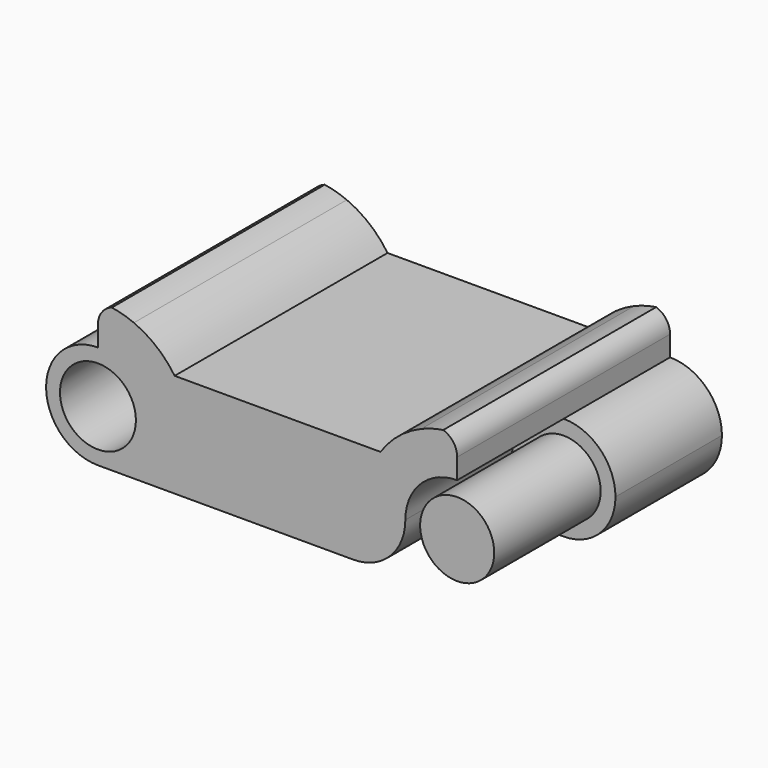
from build123d import *

# Parameters (mm, degrees)
F1_DEPTH = 14.37
F0_R     = 2
F2_DEPTH = 7.185
F3_R     = 2.05
F4_DEPTH = 7.185


with BuildPart() as f1:
    # F0 (on Front) → F1 (new body)
    with BuildSketch(Plane.XZ):
        with BuildLine():
            ThreePointArc((7.1321428571, 0.3034947896), (7.7481620558, 0.0769305381), (8.4, 0))
            Line((8.4, 0), (16.6, 0))
            ThreePointArc((16.6, 0), (17.2518379442, 0.0769305381), (17.8678571429, 0.3034947896))
            ThreePointArc((17.8678571429, 0.3034947896), (18.9864199128, 1.3354181484), (19.4, 2.8))
            ThreePointArc((19.4, 2.8), (20.2201010127, 4.7798989873), (22.2, 5.6))
            Line((22.2, 5.6), (22.2, 6.7))
            ThreePointArc((22.2, 6.7), (21.8778174593, 5.9221825407), (21.1, 5.6))
            Line((21.1, 5.6), (18.0575369646, 5.6))
            Line((18.0575369646, 5.6), (6.9424630354, 5.6))
            Line((6.9424630354, 5.6), (3.9, 5.6))
            Line((3.9, 5.6), (2.8, 5.6))
            ThreePointArc((2.8, 5.6), (4.7798989873, 4.7798989873), (5.6, 2.8))
            ThreePointArc((5.6, 2.8), (6.0135800872, 1.3354181484), (7.1321428571, 0.3034947896))
        make_face()
        with BuildLine():
            ThreePointArc((20.2574998019, 7.4072435339), (19.0261653027, 6.6635182559), (18.0575369646, 5.6))
            Line((18.0575369646, 5.6), (21.1, 5.6))
            ThreePointArc((21.1, 5.6), (20.103012566, 6.2352247249), (20.2574998019, 7.4072435339))
        make_face()
        with BuildLine():
            ThreePointArc((20.2574998019, 7.4072435339), (20.103012566, 6.2352247249), (21.1, 5.6))
            ThreePointArc((21.1, 5.6), (21.8778174593, 5.9221825407), (22.2, 6.7))
            ThreePointArc((22.2, 6.7), (21.9926506427, 7.3427867688), (21.4487730361, 7.7432436768))
            ThreePointArc((21.4487730361, 7.7432436768), (20.8426991749, 7.6122483799), (20.2574998019, 7.4072435339))
        make_face()
        with BuildLine():
            ThreePointArc((4.7425001981, 7.4072435339), (4.896987434, 6.2352247249), (3.9, 5.6))
            Line((3.9, 5.6), (6.9424630354, 5.6))
            ThreePointArc((6.9424630354, 5.6), (5.9738346973, 6.6635182559), (4.7425001981, 7.4072435339))
        make_face()
        with BuildLine():
            ThreePointArc((2.8, 6.7), (3.1221825407, 5.9221825407), (3.9, 5.6))
            ThreePointArc((3.9, 5.6), (4.896987434, 6.2352247249), (4.7425001981, 7.4072435339))
            ThreePointArc((4.7425001981, 7.4072435339), (4.1573008251, 7.6122483799), (3.5512269639, 7.7432436768))
            ThreePointArc((3.5512269639, 7.7432436768), (3.0073493573, 7.3427867688), (2.8, 6.7))
        make_face()
        with BuildLine():
            Line((2.8, 6.7), (2.8, 5.6))
            Line((2.8, 5.6), (3.9, 5.6))
            ThreePointArc((3.9, 5.6), (3.1221825407, 5.9221825407), (2.8, 6.7))
        make_face()
    extrude(amount=F1_DEPTH)



with BuildPart() as f1b:
    # F0 (on Front) → F1, piece 2 (new body)
    with BuildSketch(Plane.XZ):
        with Locations((22.2, 2.8)):
            Circle(F0_R)
    extrude(amount=F1_DEPTH)


with BuildPart() as f1_1:
    add(f1.part)

    add(f1b.part)  # F2 merges F1b
    # F0 (on Front) → F2 (join)
    with BuildSketch(Plane.XZ):
        with BuildLine():
            ThreePointArc((17.8678571429, 0.3034947896), (17.2518379442, 0.0769305381), (16.6, 0))
            Line((16.6, 0), (22.2, 0))
            ThreePointArc((22.2, 0), (20.2201010127, 0.8201010127), (19.4, 2.8))
            ThreePointArc((19.4, 2.8), (18.9864199128, 1.3354181484), (17.8678571429, 0.3034947896))
        make_face()
        with BuildLine():
            ThreePointArc((19.4, 2.8), (20.2201010127, 0.8201010127), (22.2, 0))
            ThreePointArc((22.2, 0), (24.1798989873, 0.8201010127), (25, 2.8))
            ThreePointArc((25, 2.8), (24.1798989873, 4.7798989873), (22.2, 5.6))
            ThreePointArc((22.2, 5.6), (20.2201010127, 4.7798989873), (19.4, 2.8))
        make_face()
        with Locations((22.2, 2.8)):
            Circle(F0_R, mode=Mode.SUBTRACT)
    extrude(amount=F2_DEPTH)

    # F3 (on face) → F4 (join)
    with BuildSketch(Plane.XZ.offset(14.37)):
        with BuildLine():
            ThreePointArc((2.8, 0), (4.7798989873, 0.8201010127), (5.6, 2.8))
            ThreePointArc((5.6, 2.8), (4.7798989873, 4.7798989873), (2.8, 5.6))
            ThreePointArc((2.8, 5.6), (0, 2.8), (2.8, 0))
        make_face()
        with Locations((2.8, 2.8)):
            Circle(F3_R, mode=Mode.SUBTRACT)
        with BuildLine():
            ThreePointArc((8.4, 0), (6.4201010127, 0.8201010127), (5.6, 2.8))
            ThreePointArc((5.6, 2.8), (4.7798989873, 0.8201010127), (2.8, 0))
            Line((2.8, 0), (8.4, 0))
        make_face()
    extrude(amount=-F4_DEPTH)


solid = f1_1.part
